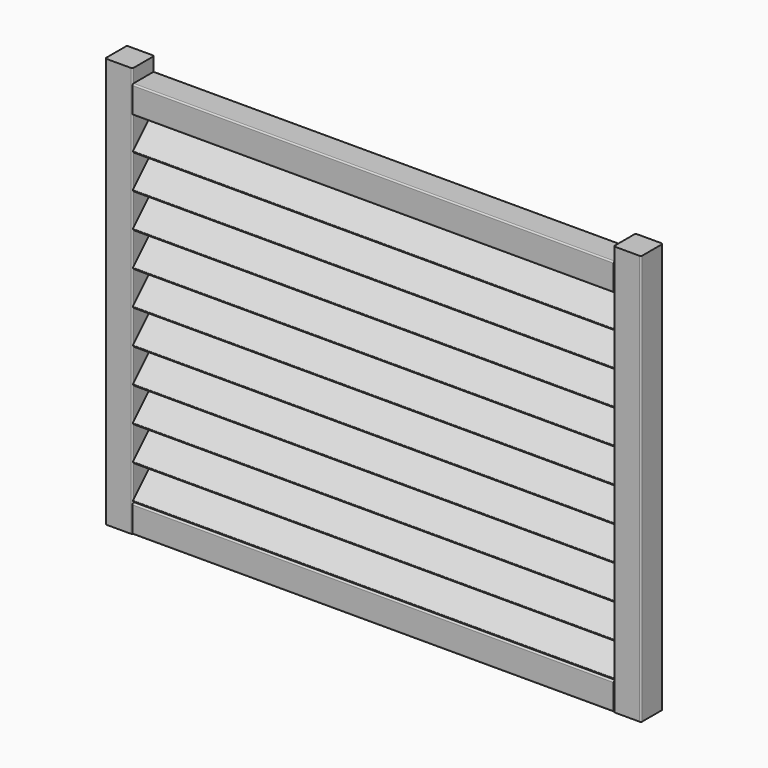
from build123d import *

# Parameters (mm, degrees)
F1_DEPTH      = 1760
F3_DEPTH      = 1400
F3_DEPTH_BACK = 100
F4_W          = 90
F4_H          = 100
F5_DEPTH      = 1760


# Not quite as in the source:
# - a feature names something its author has since deleted; it is built from what else it names


with BuildPart() as f1:
    # F0 (on Right) → F1 (new body)
    with BuildSketch(Plane.YZ):
        with BuildLine():
            ThreePointArc((-1.4142135624, 1.4142135624), (0, 0.8284271247), (1.4142135624, 1.4142135624))
            Line((1.4142135624, 1.4142135624), (89.8025612107, 89.8025612107))
            ThreePointArc((89.8025612107, 89.8025612107), (90.3883476483, 91.2167747731), (89.8025612107, 92.6309883354))
            Line((89.8025612107, 92.6309883354), (85.5599205236, 96.8736290226))
            ThreePointArc((85.5599205236, 96.8736290226), (84.1457069612, 97.4594154602), (82.7314933988, 96.8736290226))
            Line((82.7314933988, 96.8736290226), (-5.6568542495, 8.4852813742))
            ThreePointArc((-5.6568542495, 8.4852813742), (-6.2426406871, 7.0710678119), (-5.6568542495, 5.6568542495))
            Line((-5.6568542495, 5.6568542495), (-1.4142135624, 1.4142135624))
        make_face()
    extrude(amount=F1_DEPTH)


with BuildPart() as f1b:
    # F0 (on Right) → F1, piece 2 (new body)
    with BuildSketch(Plane.YZ):
        with BuildLine():
            ThreePointArc((-1.4142135624, 126.4142135624), (0, 125.8284271247), (1.4142135624, 126.4142135624))
            Line((1.4142135624, 126.4142135624), (89.8025612107, 214.8025612107))
            ThreePointArc((89.8025612107, 214.8025612107), (90.3883476483, 216.2167747731), (89.8025612107, 217.6309883354))
            Line((89.8025612107, 217.6309883354), (85.5599205236, 221.8736290226))
            ThreePointArc((85.5599205236, 221.8736290226), (84.1457069612, 222.4594154602), (82.7314933988, 221.8736290226))
            Line((82.7314933988, 221.8736290226), (-5.6568542495, 133.4852813742))
            ThreePointArc((-5.6568542495, 133.4852813742), (-6.2426406871, 132.0710678119), (-5.6568542495, 130.6568542495))
            Line((-5.6568542495, 130.6568542495), (-1.4142135624, 126.4142135624))
        make_face()
    extrude(amount=F1_DEPTH)


with BuildPart() as f1c:
    # F0 (on Right) → F1, piece 3 (new body)
    with BuildSketch(Plane.YZ):
        with BuildLine():
            ThreePointArc((-1.4142135624, 251.4142135624), (0, 250.8284271247), (1.4142135624, 251.4142135624))
            Line((1.4142135624, 251.4142135624), (89.8025612107, 339.8025612107))
            ThreePointArc((89.8025612107, 339.8025612107), (90.3883476483, 341.2167747731), (89.8025612107, 342.6309883354))
            Line((89.8025612107, 342.6309883354), (85.5599205236, 346.8736290226))
            ThreePointArc((85.5599205236, 346.8736290226), (84.1457069612, 347.4594154602), (82.7314933988, 346.8736290226))
            Line((82.7314933988, 346.8736290226), (-5.6568542495, 258.4852813742))
            ThreePointArc((-5.6568542495, 258.4852813742), (-6.2426406871, 257.0710678119), (-5.6568542495, 255.6568542495))
            Line((-5.6568542495, 255.6568542495), (-1.4142135624, 251.4142135624))
        make_face()
    extrude(amount=F1_DEPTH)


with BuildPart() as f1d:
    # F0 (on Right) → F1, piece 4 (new body)
    with BuildSketch(Plane.YZ):
        with BuildLine():
            ThreePointArc((-1.4142135624, 376.4142135624), (0, 375.8284271247), (1.4142135624, 376.4142135624))
            Line((1.4142135624, 376.4142135624), (89.8025612107, 464.8025612107))
            ThreePointArc((89.8025612107, 464.8025612107), (90.3883476483, 466.2167747731), (89.8025612107, 467.6309883354))
            Line((89.8025612107, 467.6309883354), (85.5599205236, 471.8736290226))
            ThreePointArc((85.5599205236, 471.8736290226), (84.1457069612, 472.4594154602), (82.7314933988, 471.8736290226))
            Line((82.7314933988, 471.8736290226), (-5.6568542495, 383.4852813742))
            ThreePointArc((-5.6568542495, 383.4852813742), (-6.2426406871, 382.0710678119), (-5.6568542495, 380.6568542495))
            Line((-5.6568542495, 380.6568542495), (-1.4142135624, 376.4142135624))
        make_face()
    extrude(amount=F1_DEPTH)


with BuildPart() as f1e:
    # F0 (on Right) → F1, piece 5 (new body)
    with BuildSketch(Plane.YZ):
        with BuildLine():
            ThreePointArc((-1.4142135624, 501.4142135624), (0, 500.8284271247), (1.4142135624, 501.4142135624))
            Line((1.4142135624, 501.4142135624), (89.8025612107, 589.8025612107))
            ThreePointArc((89.8025612107, 589.8025612107), (90.3883476483, 591.2167747731), (89.8025612107, 592.6309883354))
            Line((89.8025612107, 592.6309883354), (85.5599205236, 596.8736290226))
            ThreePointArc((85.5599205236, 596.8736290226), (84.1457069612, 597.4594154602), (82.7314933988, 596.8736290226))
            Line((82.7314933988, 596.8736290226), (-5.6568542495, 508.4852813742))
            ThreePointArc((-5.6568542495, 508.4852813742), (-6.2426406871, 507.0710678119), (-5.6568542495, 505.6568542495))
            Line((-5.6568542495, 505.6568542495), (-1.4142135624, 501.4142135624))
        make_face()
    extrude(amount=F1_DEPTH)


with BuildPart() as f1f:
    # F0 (on Right) → F1, piece 6 (new body)
    with BuildSketch(Plane.YZ):
        with BuildLine():
            ThreePointArc((-1.4142135624, 626.4142135624), (0, 625.8284271247), (1.4142135624, 626.4142135624))
            Line((1.4142135624, 626.4142135624), (89.8025612107, 714.8025612107))
            ThreePointArc((89.8025612107, 714.8025612107), (90.3883476483, 716.2167747731), (89.8025612107, 717.6309883354))
            Line((89.8025612107, 717.6309883354), (85.5599205236, 721.8736290226))
            ThreePointArc((85.5599205236, 721.8736290226), (84.1457069612, 722.4594154602), (82.7314933988, 721.8736290226))
            Line((82.7314933988, 721.8736290226), (-5.6568542495, 633.4852813742))
            ThreePointArc((-5.6568542495, 633.4852813742), (-6.2426406871, 632.0710678119), (-5.6568542495, 630.6568542495))
            Line((-5.6568542495, 630.6568542495), (-1.4142135624, 626.4142135624))
        make_face()
    extrude(amount=F1_DEPTH)


with BuildPart() as f1g:
    # F0 (on Right) → F1, piece 7 (new body)
    with BuildSketch(Plane.YZ):
        with BuildLine():
            ThreePointArc((-1.4142135624, 751.4142135624), (0, 750.8284271247), (1.4142135624, 751.4142135624))
            Line((1.4142135624, 751.4142135624), (89.8025612107, 839.8025612107))
            ThreePointArc((89.8025612107, 839.8025612107), (90.3883476483, 841.2167747731), (89.8025612107, 842.6309883354))
            Line((89.8025612107, 842.6309883354), (85.5599205236, 846.8736290226))
            ThreePointArc((85.5599205236, 846.8736290226), (84.1457069612, 847.4594154602), (82.7314933988, 846.8736290226))
            Line((82.7314933988, 846.8736290226), (-5.6568542495, 758.4852813742))
            ThreePointArc((-5.6568542495, 758.4852813742), (-6.2426406871, 757.0710678119), (-5.6568542495, 755.6568542495))
            Line((-5.6568542495, 755.6568542495), (-1.4142135624, 751.4142135624))
        make_face()
    extrude(amount=F1_DEPTH)


with BuildPart() as f1h:
    # F0 (on Right) → F1, piece 8 (new body)
    with BuildSketch(Plane.YZ):
        with BuildLine():
            ThreePointArc((-1.4142135624, 876.4142135624), (0, 875.8284271247), (1.4142135624, 876.4142135624))
            Line((1.4142135624, 876.4142135624), (89.8025612107, 964.8025612107))
            ThreePointArc((89.8025612107, 964.8025612107), (90.3883476483, 966.2167747731), (89.8025612107, 967.6309883354))
            Line((89.8025612107, 967.6309883354), (85.5599205236, 971.8736290226))
            ThreePointArc((85.5599205236, 971.8736290226), (84.1457069612, 972.4594154602), (82.7314933988, 971.8736290226))
            Line((82.7314933988, 971.8736290226), (-5.6568542495, 883.4852813742))
            ThreePointArc((-5.6568542495, 883.4852813742), (-6.2426406871, 882.0710678119), (-5.6568542495, 880.6568542495))
            Line((-5.6568542495, 880.6568542495), (-1.4142135624, 876.4142135624))
        make_face()
    extrude(amount=F1_DEPTH)


with BuildPart() as f1i:
    # F0 (on Right) → F1, piece 9 (new body)
    with BuildSketch(Plane.YZ):
        with BuildLine():
            ThreePointArc((-1.4142135624, 1001.4142135624), (0, 1000.8284271247), (1.4142135624, 1001.4142135624))
            Line((1.4142135624, 1001.4142135624), (89.8025612107, 1089.8025612107))
            ThreePointArc((89.8025612107, 1089.8025612107), (90.3883476483, 1091.2167747731), (89.8025612107, 1092.6309883354))
            Line((89.8025612107, 1092.6309883354), (85.5599205236, 1096.8736290226))
            ThreePointArc((85.5599205236, 1096.8736290226), (84.1457069612, 1097.4594154602), (82.7314933988, 1096.8736290226))
            Line((82.7314933988, 1096.8736290226), (-5.6568542495, 1008.4852813742))
            ThreePointArc((-5.6568542495, 1008.4852813742), (-6.2426406871, 1007.0710678119), (-5.6568542495, 1005.6568542495))
            Line((-5.6568542495, 1005.6568542495), (-1.4142135624, 1001.4142135624))
        make_face()
    extrude(amount=F1_DEPTH)


with BuildPart() as f1j:
    # F0 (on Right) → F1, piece 10 (new body)
    with BuildSketch(Plane.YZ):
        with BuildLine():
            ThreePointArc((-1.4142135624, 1126.4142135624), (0, 1125.8284271247), (1.4142135624, 1126.4142135624))
            Line((1.4142135624, 1126.4142135624), (89.8025612107, 1214.8025612107))
            ThreePointArc((89.8025612107, 1214.8025612107), (90.3883476483, 1216.2167747731), (89.8025612107, 1217.6309883354))
            Line((89.8025612107, 1217.6309883354), (85.5599205236, 1221.8736290226))
            ThreePointArc((85.5599205236, 1221.8736290226), (84.1457069612, 1222.4594154602), (82.7314933988, 1221.8736290226))
            Line((82.7314933988, 1221.8736290226), (-5.6568542495, 1133.4852813742))
            ThreePointArc((-5.6568542495, 1133.4852813742), (-6.2426406871, 1132.0710678119), (-5.6568542495, 1130.6568542495))
            Line((-5.6568542495, 1130.6568542495), (-1.4142135624, 1126.4142135624))
        make_face()
    extrude(amount=F1_DEPTH)


with BuildPart() as f3:
    # F2 (on Top) → F3 (new body, two sides)
    with BuildSketch(Plane.XY) as f3_sk:
        with BuildLine():
            Line((-95, -8), (-5, -8))
            ThreePointArc((-5, -8), (-1.4644660941, -6.5355339059), (0, -3))
            Line((0, -3), (0, 87))
            ThreePointArc((0, 87), (-1.4644660941, 90.5355339059), (-5, 92))
            Line((-5, 92), (-95, 92))
            ThreePointArc((-95, 92), (-98.5355339059, 90.5355339059), (-100, 87))
            Line((-100, 87), (-100, -3))
            ThreePointArc((-100, -3), (-98.5355339059, -6.5355339059), (-95, -8))
        make_face()
    extrude(amount=F3_DEPTH)
    extrude(f3_sk.sketch, amount=-F3_DEPTH_BACK)


with BuildPart() as f3b:
    # F2 (on Top) → F3, piece 2 (new body, two sides)
    with BuildSketch(Plane.XY) as f3_2_sk:
        with BuildLine():
            Line((1760, 87), (1760, -3))
            ThreePointArc((1760, -3), (1761.4644660941, -6.5355339059), (1765, -8))
            Line((1765, -8), (1855, -8))
            ThreePointArc((1855, -8), (1858.5355339059, -6.5355339059), (1860, -3))
            Line((1860, -3), (1860, 87))
            ThreePointArc((1860, 87), (1858.5355339059, 90.5355339059), (1855, 92))
            Line((1855, 92), (1765, 92))
            ThreePointArc((1765, 92), (1761.4644660941, 90.5355339059), (1760, 87))
        make_face()
    extrude(amount=F3_DEPTH)
    extrude(f3_2_sk.sketch, amount=-F3_DEPTH_BACK)


with BuildPart() as f5:
    # F4 (on face) → F5 (new body)
    with BuildSketch(Plane.YZ):
        with Locations((42, 1300)):
            Rectangle(F4_W, F4_H)
        with BuildLine():
            ThreePointArc((-8, 1255), (-6.5355339059, 1251.4644660941), (-3, 1250))
            Line((-3, 1250), (-3, 1350))
            ThreePointArc((-3, 1350), (-6.5355339059, 1348.5355339059), (-8, 1345))
            Line((-8, 1345), (-8, 1255))
        make_face()
        with BuildLine():
            Line((87, 1350), (87, 1250))
            ThreePointArc((87, 1250), (90.5355339059, 1251.4644660941), (92, 1255))
            Line((92, 1255), (92, 1345))
            ThreePointArc((92, 1345), (90.5355339059, 1348.5355339059), (87, 1350))
        make_face()
    extrude(amount=F5_DEPTH)


with BuildPart() as f5b:
    # F4 (on face) → F5, piece 2 (new body)
    with BuildSketch(Plane.YZ):
        with Locations((42, -50)):
            Rectangle(F4_W, F4_H)
        with BuildLine():
            ThreePointArc((-8, -95), (-6.5355339059, -98.5355339059), (-3, -100))
            Line((-3, -100), (-3, 0))
            ThreePointArc((-3, 0), (-6.5355339059, -1.4644660941), (-8, -5))
            Line((-8, -5), (-8, -95))
        make_face()
        with BuildLine():
            Line((87, 0), (87, -100))
            ThreePointArc((87, -100), (90.5355339059, -98.5355339059), (92, -95))
            Line((92, -95), (92, -5))
            ThreePointArc((92, -5), (90.5355339059, -1.4644660941), (87, 0))
        make_face()
    extrude(amount=F5_DEPTH)


solid = Compound([f1.part, f1b.part, f1c.part, f1d.part, f1e.part, f1f.part, f1g.part, f1h.part, f1i.part, f1j.part, f3.part, f3b.part, f5.part, f5b.part])
